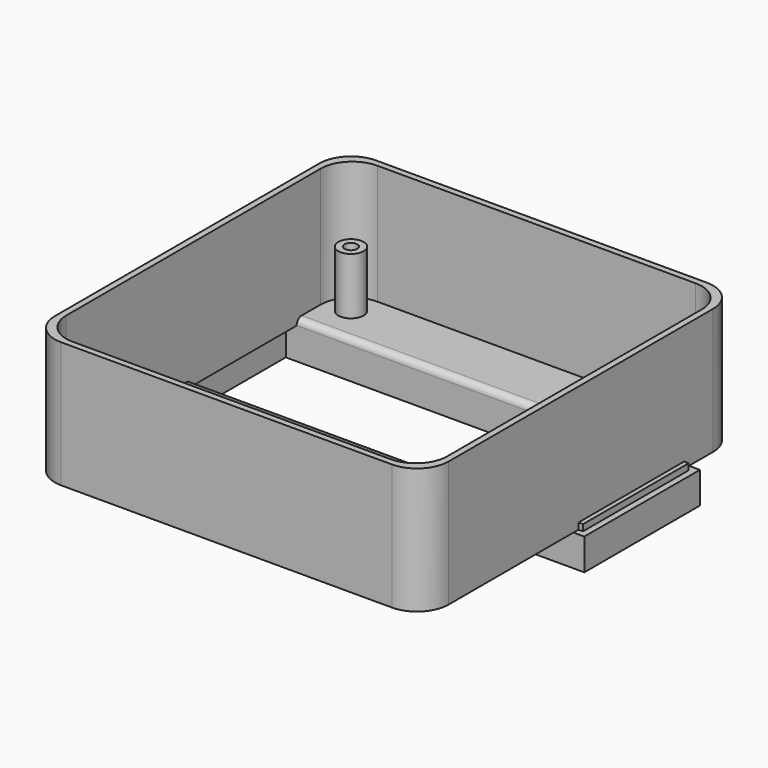
from build123d import *

# Parameters (mm, degrees)
F0_W     = 121
F0_H     = 17.55
F0_R     = 4
F0_H_2   = 2
F1_DEPTH = 2
F0_H_3   = 57.55
F0_W_2   = 1.45
F0_H_4   = 41.9
F0_W_3   = 2
F2_DEPTH = 40
F0_R_2   = 2
F3_DEPTH = 20
F4_DEPTH = 10
F5_R     = 10
F6_R     = 1.99999
F6_2_R   = 1.99999
F7_R     = 5
F7_2_R   = 5


# Not quite as in the source:
# - a fillet or chamfer is up to 0.001 mm smaller than in the source, because OpenCascade refuses the exact size


with BuildPart() as f1:
    # F0 (on Top) → F1 (new body)
    with BuildSketch(Plane.XY):
        with Locations((0, 51.725)):
            Rectangle(F0_W, F0_H)
        with Locations((-52.5, 52.5)):
            Circle(F0_R, mode=Mode.SUBTRACT)
        with Locations((52.5, 52.5)):
            Circle(F0_R, mode=Mode.SUBTRACT)
        with Locations((0, 41.95)):
            Rectangle(F0_W, F0_H_2)
    extrude(amount=F1_DEPTH)

    # F6#2 (radius 2 in the source; OpenCascade refuses exactly that, so slightly less here)
    f6_2_edges = [f1.edges().sort_by_distance(p)[0] for p in [
        (0, 40.95, 2),
    ]]
    fillet(f6_2_edges, radius=F6_2_R)

    # F7
    f7_edges = [f1.edges().sort_by_distance(p)[0] for p in [
        (60.5, 60.5, 1),
        (-60.5, 60.5, 1),
    ]]
    fillet(f7_edges, radius=F7_R)


with BuildPart() as f1b:
    # F0 (on Top) → F1, piece 2 (new body)
    with BuildSketch(Plane.XY):
        with Locations((0, -31.725)):
            Rectangle(F0_W, F0_H_3)
        with Locations((-52.5, -52.5)):
            Circle(F0_R, mode=Mode.SUBTRACT)
        with Locations((52.5, -52.5)):
            Circle(F0_R, mode=Mode.SUBTRACT)
        with Locations((0, -1.95)):
            Rectangle(F0_W, F0_H_2)
    extrude(amount=F1_DEPTH)

    # F6 (radius 2 in the source; OpenCascade refuses exactly that, so slightly less here)
    f6_edges = [f1b.edges().sort_by_distance(p)[0] for p in [
        (0, -0.95, 2),
    ]]
    fillet(f6_edges, radius=F6_R)

    # F7#2
    f7_2_edges = [f1b.edges().sort_by_distance(p)[0] for p in [
        (-60.5, -60.5, 1),
        (60.5, -60.5, 1),
    ]]
    fillet(f7_2_edges, radius=F7_2_R)


with BuildPart() as f1c:
    # F0 (on Top) → F1, piece 3 (new body)
    with BuildSketch(Plane.XY):
        with Locations((-63.225, 20)):
            Rectangle(F0_W_2, F0_H_4)
    extrude(amount=F1_DEPTH)


with BuildPart() as f1d:
    # F0 (on Top) → F1, piece 4 (new body)
    with BuildSketch(Plane.XY):
        with Locations((63.225, 20)):
            Rectangle(F0_W_2, F0_H_4)
    extrude(amount=F1_DEPTH)


with BuildPart() as f2:
    # F0 (on Top) → F2 (new body)
    with BuildSketch(Plane.XY):
        Polygon((60.5, 60.5), (60.5, 42.95), (62.5, 42.95), (62.5, 62.5), (-62.5, 62.5), (-62.5, 42.95), (-60.5, 42.95), (-60.5, 60.5), align=None)
        with Locations((-61.5, 41.95)):
            Rectangle(F0_W_3, F0_H_2)
        with Locations((-61.5, 20)):
            Rectangle(F0_W_3, F0_H_4)
        Polygon((60.5, -2.95), (60.5, -60.5), (-60.5, -60.5), (-60.5, -2.95), (-62.5, -2.95), (-62.5, -62.5), (62.5, -62.5), (62.5, -2.95), align=None)
        with Locations((-61.5, -1.95)):
            Rectangle(F0_W_3, F0_H_2)
        with Locations((61.5, -1.95)):
            Rectangle(F0_W_3, F0_H_2)
        with Locations((61.5, 20)):
            Rectangle(F0_W_3, F0_H_4)
        with Locations((61.5, 41.95)):
            Rectangle(F0_W_3, F0_H_2)
    extrude(amount=F2_DEPTH)

    # F5
    f5_edges = [f2.edges().sort_by_distance(p)[0] for p in [
        (-60.5, 60.5, 20),
        (60.5, 60.5, 20),
        (-60.5, -60.5, 20),
        (60.5, -60.5, 20),
        (-62.5, 62.5, 20),
        (62.5, 62.5, 20),
        (62.5, -62.5, 20),
        (-62.5, -62.5, 20),
    ]]
    fillet(f5_edges, radius=F5_R)


with BuildPart() as f3:
    # F0 (on Top) → F3 (new body)
    with BuildSketch(Plane.XY):
        with Locations((-52.5, 52.5)):
            Circle(F0_R)
        with Locations((-52.5, 52.5)):
            Circle(F0_R_2, mode=Mode.SUBTRACT)
    extrude(amount=F3_DEPTH)


with BuildPart() as f3b:
    # F0 (on Top) → F3, piece 2 (new body)
    with BuildSketch(Plane.XY):
        with Locations((52.5, 52.5)):
            Circle(F0_R)
        with Locations((52.5, 52.5)):
            Circle(F0_R_2, mode=Mode.SUBTRACT)
    extrude(amount=F3_DEPTH)


with BuildPart() as f3c:
    # F0 (on Top) → F3, piece 3 (new body)
    with BuildSketch(Plane.XY):
        with Locations((52.5, -52.5)):
            Circle(F0_R)
        with Locations((52.5, -52.5)):
            Circle(F0_R_2, mode=Mode.SUBTRACT)
    extrude(amount=F3_DEPTH)


with BuildPart() as f3d:
    # F0 (on Top) → F3, piece 4 (new body)
    with BuildSketch(Plane.XY):
        with Locations((-52.5, -52.5)):
            Circle(F0_R)
        with Locations((-52.5, -52.5)):
            Circle(F0_R_2, mode=Mode.SUBTRACT)
    extrude(amount=F3_DEPTH)


with BuildPart() as f4:
    # F0 (on Top) → F4 (new body)
    with BuildSketch(Plane.XY):
        Polygon((-65.95, -2.95), (-62.5, -2.95), (-62.5, -0.95), (-63.95, -0.95), (-63.95, 40.95), (-62.5, 40.95), (-62.5, 42.95), (-65.95, 42.95), align=None)
        with Locations((-61.5, -1.95)):
            Rectangle(F0_W_3, F0_H_2)
        with Locations((-61.5, 41.95)):
            Rectangle(F0_W_3, F0_H_2)
        with Locations((0, -1.95)):
            Rectangle(F0_W, F0_H_2)
        with Locations((0, 41.95)):
            Rectangle(F0_W, F0_H_2)
        with Locations((61.5, -1.95)):
            Rectangle(F0_W_3, F0_H_2)
        with Locations((61.5, 41.95)):
            Rectangle(F0_W_3, F0_H_2)
        Polygon((62.5, -0.95), (62.5, -2.95), (65.95, -2.95), (65.95, 42.95), (62.5, 42.95), (62.5, 40.95), (63.95, 40.95), (63.95, -0.95), align=None)
    extrude(amount=-F4_DEPTH)


solid = Compound([f1.part, f1b.part, f1c.part, f1d.part, f2.part, f3.part, f3b.part, f3c.part, f3d.part, f4.part])
